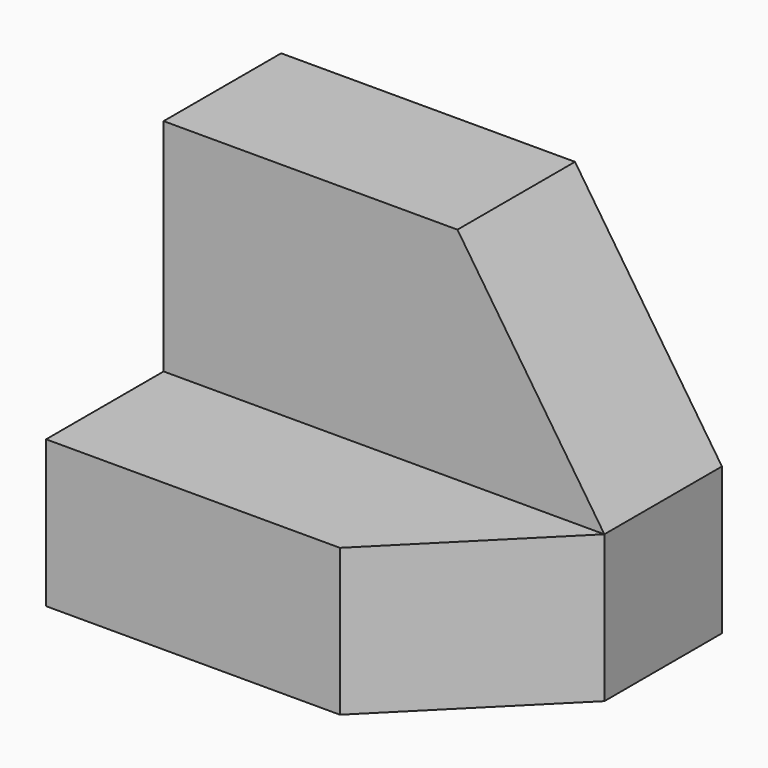
from build123d import *

# Parameters (mm, degrees)
F0_W     = 38.1
F0_H     = 31.75
F1_DEPTH = 25.4
F2_W     = 12.7
F2_H     = 19.05
F3_DEPTH = 38.1
F5_DEPTH = 12.7
F7_DEPTH = 12.7


# Not quite as in the source:
# - a length typed as a fraction of an inch, garbled in the dataset ("3 / 203.2 mm" for 3/8 in), is restored


with BuildPart() as f1:
    # F0 (on Front) → F1 (new body)
    with BuildSketch(Plane.XZ):
        with Locations((19.05, 15.875)):
            Rectangle(F0_W, F0_H)
    extrude(amount=F1_DEPTH)

    # F2 (on face) → F3 (cut)
    with BuildSketch(Plane.YZ.offset(38.1)):
        with Locations((-19.05, 22.225)):
            Rectangle(F2_W, F2_H)
    extrude(amount=-F3_DEPTH, mode=Mode.SUBTRACT)

    # F4 (on face) → F5 (cut)
    with BuildSketch(Plane(origin=(0, 0, 0), x_dir=(1, 0, 0), z_dir=(0, 0, -1))):
        Polygon((38.1, 25.4), (25.4, 25.4), (38.1, 12.7), align=None)
    extrude(amount=-F5_DEPTH, mode=Mode.SUBTRACT)

    # F6 (on face) → F7 (cut)
    with BuildSketch(Plane.XZ.offset(12.7)):
        Polygon((38.1, 31.75), (25.4, 31.75), (38.1, 12.7), align=None)
    extrude(amount=-F7_DEPTH, mode=Mode.SUBTRACT)


solid = f1.part
